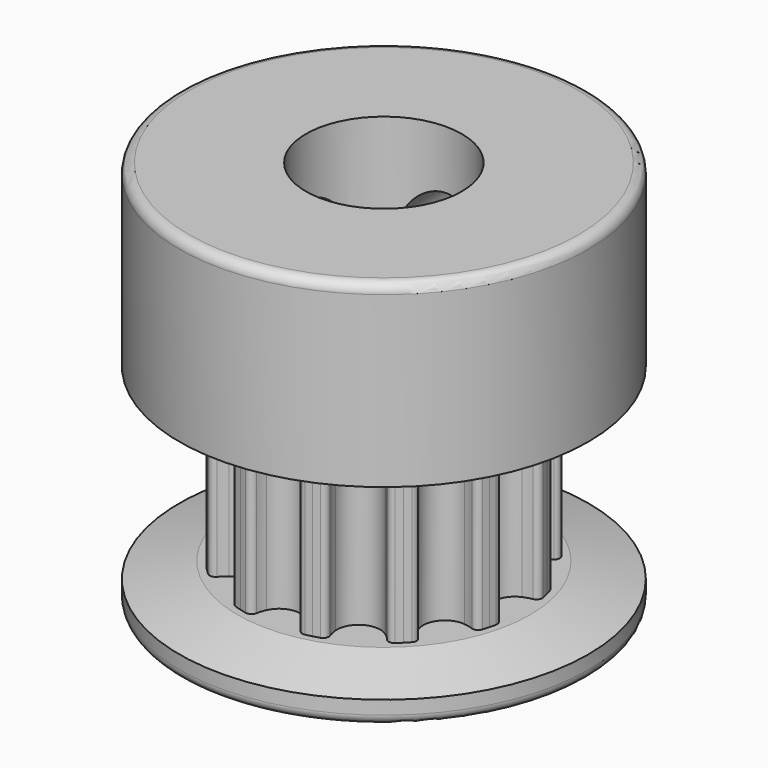
from build123d import *

# Parameters (mm, degrees)
F3_DEPTH    = 2
F4_COUNT    = 12
F5_R        = 5.25
F6_DEPTH    = 1
F7_R        = 5.25
F8_DEPTH    = 1
F9_R        = 5.25
F10_DEPTH   = 4
F11_R       = 2
F12_DEPTH   = 10.001
F13_R       = 1
F14_DEPTH   = 5.251
F15_R       = 1
F16_DEPTH   = 5.2510001
F17_SIZE2   = 0.4019237886
F17_SIZE    = 1.5
F17_2_SIZE2 = 0.4019237886
F17_2_SIZE  = 1.5
F18_R       = 0.25


# Not quite as in the source:
# - a feature names something its author has since deleted; it is built from what else it names


with BuildPart() as f3:
    # F2 (on Top) → F3 (new body, symmetric)
    with BuildSketch(Plane.XY):
        with BuildLine():
            ThreePointArc((0.506505233, 3.1337114797), (0.3017474401, 2.8947937783), (0, 2.8055979028))
            ThreePointArc((0, 2.8055979028), (-0.3017474401, 2.8947937783), (-0.506505233, 3.1337114797))
            ThreePointArc((-0.506505233, 3.1337114797), (-0.549200471, 3.2469335464), (-0.5779078391, 3.3644835645))
            ThreePointArc((-0.5779078391, 3.3644835645), (-0.6421960545, 3.4625125609), (-0.7573721026, 3.4843560203))
            ThreePointArc((-0.7573721026, 3.4843560203), (-0.8403636484, 3.4652760809), (-0.922875892, 3.4442197181))
            Line((-0.922875892, 3.4442197181), (0, 0))
            Line((0, 0), (0.922875892, 3.4442197181))
            ThreePointArc((0.922875892, 3.4442197181), (0.8403636484, 3.4652760809), (0.7573721026, 3.4843560203))
            ThreePointArc((0.7573721026, 3.4843560203), (0.6421960545, 3.4625125609), (0.5779078391, 3.3644835645))
            ThreePointArc((0.5779078391, 3.3644835645), (0.549200471, 3.2469335464), (0.506505233, 3.1337114797))
        make_face()
    extrude(amount=F3_DEPTH, both=True)

    # F4: F3 ×12 about axis
    f4_axis = Axis((0, 0, 0), (0, 0, -1))


with BuildPart() as f3_1:
    add(f3.part)
    for i in range(1, F4_COUNT):
        add(f3.part.rotate(f4_axis, i * 360 / F4_COUNT))

    # F5 (on face) → F6 (join)
    with BuildSketch(Plane(origin=(0, 0, -2), x_dir=(1, 0, 0), z_dir=(0, 0, -1))):
        Circle(F5_R)
    extrude(amount=F6_DEPTH)

    # F7 (on face) → F8 (join)
    with BuildSketch(Plane.XY.offset(2)):
        Circle(F7_R)
    extrude(amount=F8_DEPTH)

    # F9 (on face) → F10 (join)
    with BuildSketch(Plane.XY.offset(3)):
        Circle(F9_R)
    extrude(amount=F10_DEPTH)

    # F11 (on face) → F12 (cut, through all)
    with BuildSketch(Plane.XY.offset(7)):
        Circle(F11_R)
    extrude(amount=-F12_DEPTH, mode=Mode.SUBTRACT)

    # F13 (on Front) → F14 (cut, through all)
    with BuildSketch(Plane.XZ):
        with Locations((0, 4.5)):
            Circle(F13_R)
    extrude(amount=-F14_DEPTH, mode=Mode.SUBTRACT)

    # F15 (on Right) → F16 (cut, through all)
    with BuildSketch(Plane.YZ):
        with Locations((0, 4.5)):
            Circle(F15_R)
    extrude(amount=-F16_DEPTH, mode=Mode.SUBTRACT)

    # F17
    f17_edges = [f3_1.edges().sort_by_distance(p)[0] for p in [
        (-5.25, 0, -2),
    ]]
    f17_side = f3_1.faces().sort_by_distance((-5.101508, 0, -2))[0]
    chamfer(f17_edges, length=F17_SIZE, length2=F17_SIZE2, reference=f17_side)

    # F17#2
    f17_2_edges = [f3_1.edges().sort_by_distance(p)[0] for p in [
        (-5.25, 0, 2),
    ]]
    f17_2_side = f3_1.faces().sort_by_distance((-5.101508, 0, 2))[0]
    chamfer(f17_2_edges, length=F17_2_SIZE, length2=F17_2_SIZE2, reference=f17_2_side)

    # F18
    f18_edges = [f3_1.edges().sort_by_distance(p)[0] for p in [
        (-5.25, 0, 7),
        (-5.25, 0, -3),
    ]]
    fillet(f18_edges, radius=F18_R)


solid = f3_1.part
